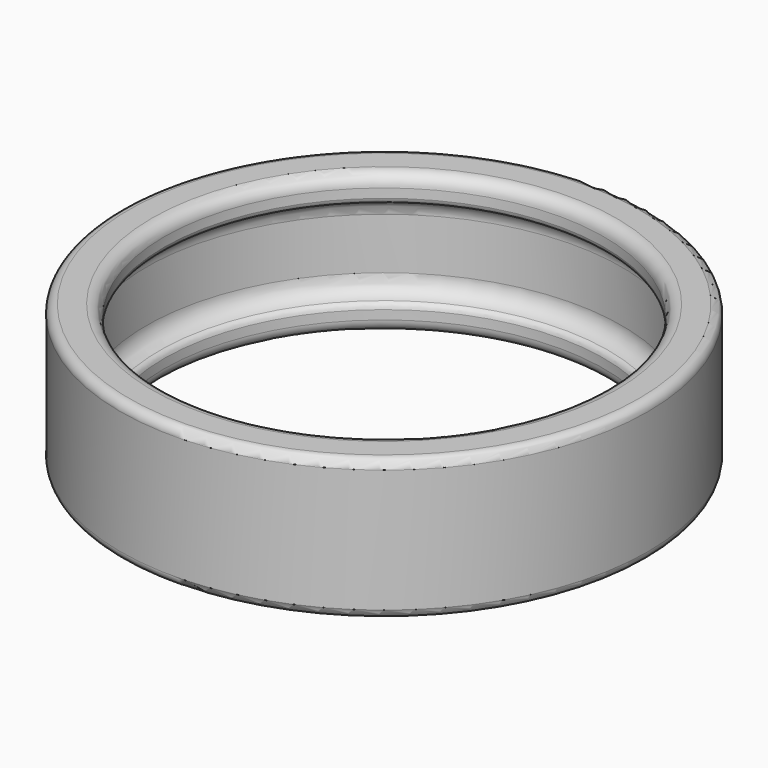
from build123d import *

# Parameters (mm, degrees)
F0_R     = 38.1
F0_R_2   = 31.75
F1_DEPTH = 10.16
F2_T     = -3.81
F3_R     = 1.778
F4_R     = 1.27
F6_R     = 0.8489579777


# Not quite as in the source:
# - a fillet or chamfer that OpenCascade refuses, or shapes differently, is made with other operations: its cross-section is extruded or revolved along the edge and cut away or added


with BuildPart() as f1:
    # F0 (on Top) → F1 (new body, symmetric)
    with BuildSketch(Plane.XY):
        Circle(F0_R)
        Circle(F0_R_2, mode=Mode.SUBTRACT)
    extrude(amount=F1_DEPTH, both=True)

    # F2
    f2_openings = [f1.faces().sort_by_distance(p)[0] for p in [
        (-31.75, 0, 0),
    ]]
    offset(amount=F2_T, openings=f2_openings)

    # F3
    f3_edges = [f1.edges().sort_by_distance(p)[0] for p in [
        (-31.75, 0, 10.16),
        (-31.75, 0, -10.16),
    ]]
    fillet(f3_edges, radius=F3_R)

    # F4
    f4_edges = [f1.edges().sort_by_distance(p)[0] for p in [
        (-38.1, 0, -10.16),
        (-38.1, 0, 10.16),
    ]]
    fillet(f4_edges, radius=F4_R)

    # F5: fillet of radius 2.6368040528 on 2 edges, made by hand

    # F5_s1 → F5_t2 (revolve)
    with BuildSketch(Plane.XZ):
        with BuildLine():
            ThreePointArc((34.29, -3.7149735128), (33.5516148856, -5.5449301098), (31.75, -6.35))
            Line((31.75, -6.35), (34.29, -6.35))
            Line((34.29, -6.35), (34.29, -3.7149735128))
        make_face()
    revolve(axis=Axis((0, 0, -6.35), (0, 0, 1)))

    # F5_s3 → F5_t4 (revolve)
    with BuildSketch(Plane.XZ):
        with BuildLine():
            ThreePointArc((31.75, 6.35), (33.5516148856, 5.5449301098), (34.29, 3.7149735128))
            Line((34.29, 3.7149735128), (34.29, 6.35))
            Line((34.29, 6.35), (31.75, 6.35))
        make_face()
    revolve(axis=Axis((0, 0, 6.35), (0, 0, 1)))

    # F6
    f6_edges = [f1.edges().sort_by_distance(p)[0] for p in [
        (-31.75, 0, 6.35),
        (-31.75, 0, -6.35),
    ]]
    fillet(f6_edges, radius=F6_R)


solid = f1.part
